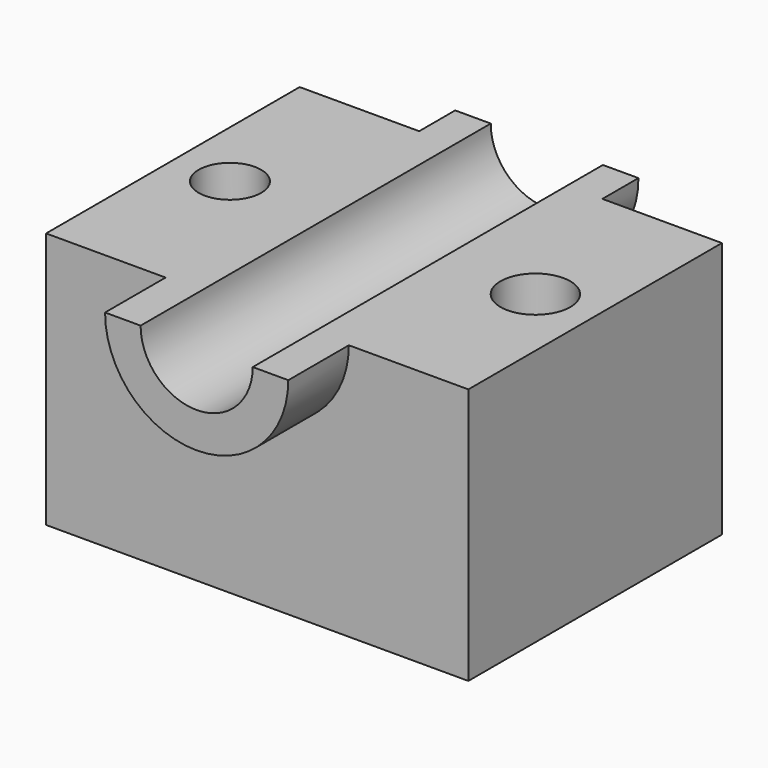
from build123d import *

# Parameters (mm, degrees)
F0_W     = 104.885712266
F0_H     = 78.7287391722
F1_DEPTH = 63.754
F3_DEPTH = 18.796
F4_DEPTH = 105.156
F5_DEPTH = 108.712
F6_R     = 7.7678468682
F6_R_2   = 8.6774880562
F7_DEPTH = 90.17


with BuildPart() as f1:
    # F0 (on Top) → F1 (new body)
    with BuildSketch(Plane.XY):
        with Locations((4.3426826596, 21.0932102054)):
            Rectangle(F0_W, F0_H)
    extrude(amount=F1_DEPTH)

    # F2 (on face) → F3 (join)
    with BuildSketch(Plane.XZ.offset(18.2711593807)):
        with BuildLine():
            Line((-9.586125523, 63.754), (-18.415103221, 63.754))
            ThreePointArc((-18.415103221, 63.754), (4.3426826596, 40.9962141193), (27.1004685403, 63.754))
            Line((27.1004685403, 63.754), (18.2714908423, 63.754))
            ThreePointArc((18.2714908423, 63.754), (4.3426826596, 49.8251918173), (-9.586125523, 63.754))
        make_face()
    extrude(amount=F3_DEPTH)

    # F4 (cut): a face of the model
    f4_faces = [f1.faces().sort_by_distance(p)[0] for p in [
        (4.3426826596, -18.2711593807, 57.8424302036),
    ]]
    extrude(f4_faces, amount=-F4_DEPTH, mode=Mode.SUBTRACT)

    # F5 (add): a face of the model
    f5_faces = [f1.faces().sort_by_distance(p)[0] for p in [
        (22.6859796913, -37.0671593807, 63.2451204375),
    ]]
    extrude(f5_faces, amount=-F5_DEPTH)

    # F6 (on face) → F7 (cut)
    with BuildSketch(Plane.XY.offset(63.754)):
        with Locations((-33.9234930099, 21.0932102054)):
            Circle(F6_R)
        with Locations((41.9430036665, 21.0932102054)):
            Circle(F6_R_2)
    extrude(amount=-F7_DEPTH, mode=Mode.SUBTRACT)


solid = f1.part
